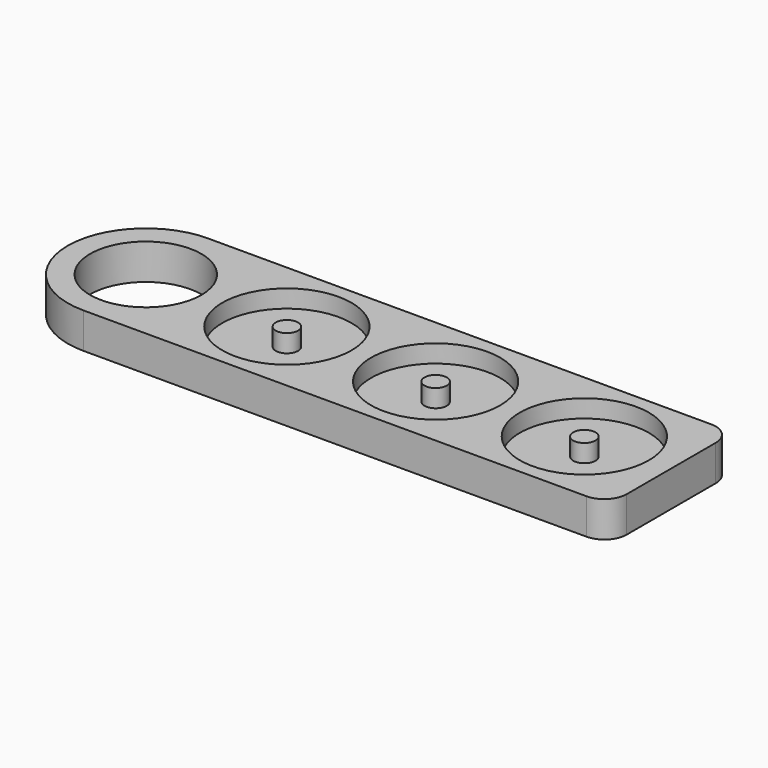
from build123d import *

# Parameters (mm, degrees)
F0_R         = 12.5
F1_DEPTH     = 8
F2_R         = 14.5
F2_R_2       = 2.5
F3_DEPTH     = 4
F4_TEXT_SIZE = 5.5555555556
F5_DEPTH     = 1


# Not quite as in the source:
# - Text() gives the source's letters only with a copy of the font that has no kerning and outlines rounded to 1/6400 em; it was checked with that copy


with BuildPart() as f1:
    # F0 (on Top) → F1 (new body)
    with BuildSketch(Plane.XY):
        with BuildLine():
            ThreePointArc((0, 17.5), (5.1256313292, 5.1256313292), (17.5, 0))
            Line((17.5, 0), (130.5, 0))
            ThreePointArc((130.5, 0), (134.0355339059, 1.4644660941), (135.5, 5))
            Line((135.5, 5), (135.5, 30))
            ThreePointArc((135.5, 30), (134.0355339059, 33.5355339059), (130.5, 35))
            Line((130.5, 35), (17.5, 35))
            ThreePointArc((17.5, 35), (5.1256313292, 29.8743686708), (0, 17.5))
        make_face()
        with Locations((17.5, 17.5)):
            Circle(F0_R, mode=Mode.SUBTRACT)
    extrude(amount=F1_DEPTH)

    # F2 (on face) → F3 (cut)
    with BuildSketch(Plane.XY.offset(8)):
        with Locations((49.2, 17.5)):
            Circle(F2_R)
        with Locations((49.2, 17.5)):
            Circle(F2_R_2, mode=Mode.SUBTRACT)
        with Locations((82.6, 17.5)):
            Circle(F2_R)
        with Locations((82.6, 17.5)):
            Circle(F2_R_2, mode=Mode.SUBTRACT)
        with Locations((116, 17.5)):
            Circle(F2_R)
        with Locations((116, 17.5)):
            Circle(F2_R_2, mode=Mode.SUBTRACT)
    extrude(amount=-F3_DEPTH, mode=Mode.SUBTRACT)

    # F4 (on face) → F5 (cut)
    with BuildSketch(Plane(origin=(0, 0, 0), x_dir=(1, 0, 0), z_dir=(0, 0, -1))):
        with Locations((30, -9)):
            Text('872', F4_TEXT_SIZE, font='Open Sans', text_align=(TextAlign.LEFT, TextAlign.BOTTOM))
    extrude(amount=-F5_DEPTH, mode=Mode.SUBTRACT)


solid = f1.part
